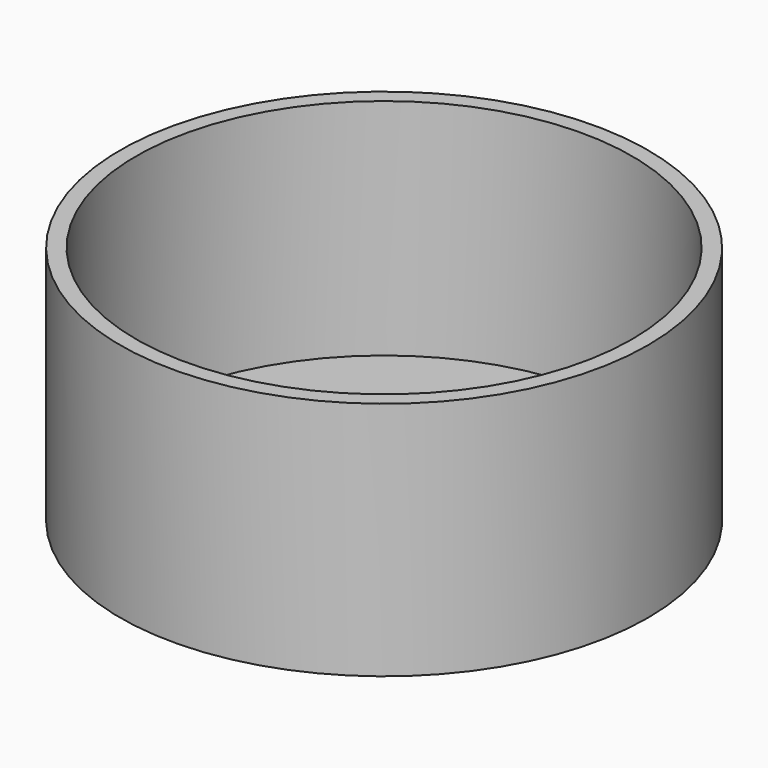
from build123d import *

# Parameters (mm, degrees)
F0_R     = 33
F1_DEPTH = 30
F2_T     = -2
F3_DEPTH = 109
F4_W     = 28
F4_H     = 28
F5_DEPTH = 12.5


# Not quite as in the source:
# - an extrude ends at something that could not be found from the text; its depth is read off the source's solid


with BuildPart() as f1:
    # F0 (on Top) → F1 (new body)
    with BuildSketch(Plane.XY):
        Circle(F0_R)
    extrude(amount=F1_DEPTH)

    # F2
    f2_openings = [f1.faces().sort_by_distance(p)[0] for p in [
        (0, 0, 30),
    ]]
    offset(amount=F2_T, openings=f2_openings)

    # F0 (on Top) → F3 (cut, through all)
    with BuildSketch(Plane.XY):
        Circle(F0_R)
    extrude(amount=-F3_DEPTH, mode=Mode.SUBTRACT)

    # F4 (on face) → F5 (cut, symmetric)
    with BuildSketch(Plane.XY):
        Rectangle(F4_W, F4_H)
    extrude(amount=F5_DEPTH, both=True, mode=Mode.SUBTRACT)


solid = f1.part
